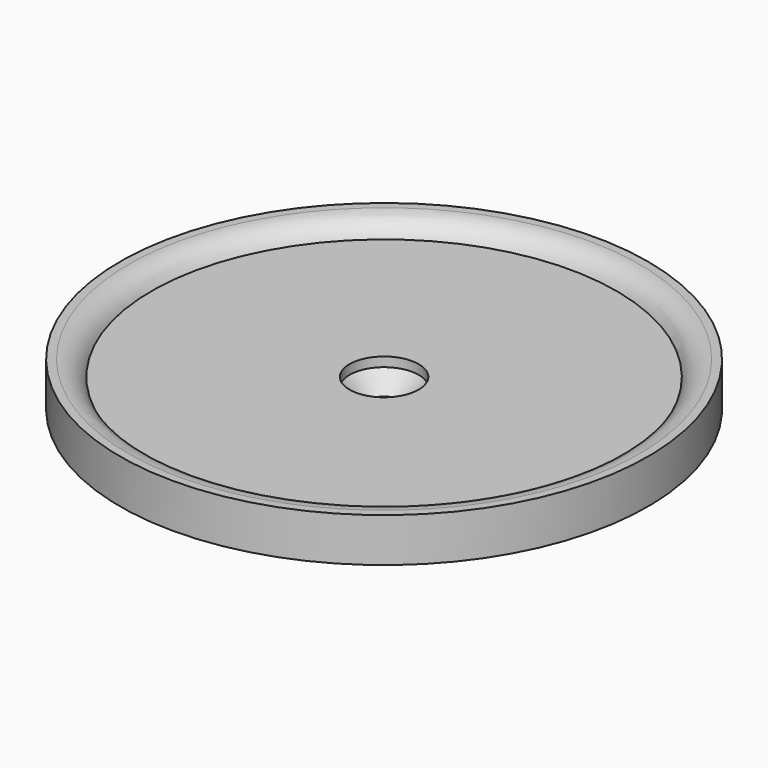
from build123d import *

# Parameters (mm, degrees)
F0_R        = 18.5
F0_R_2      = 1.4
F1_DEPTH    = 2.25
F2_R        = 2.75
F3_DEPTH    = 0.1
F4_S5_R     = 2.75
F4_T6_DEPTH = 6
F6_W        = 2.5
F6_H        = 3.5


# Not quite as in the source:
# - a fillet or chamfer that OpenCascade refuses, or shapes differently, is made with other operations: its cross-section is extruded or revolved along the edge and cut away or added
# - a feature names something its author has since deleted; it is built from what else it names


with BuildPart() as f1:
    # F0 (on Top) → F1 (new body)
    with BuildSketch(Plane.XY):
        Circle(F0_R)
        Circle(F0_R_2, mode=Mode.SUBTRACT)
    extrude(amount=F1_DEPTH)

    # F2 (on face) → F3 (cut)
    with BuildSketch(Plane.XY.offset(2.25)):
        Circle(F2_R)
    extrude(amount=-F3_DEPTH, mode=Mode.SUBTRACT)

    # F4: chamfer of 2 on 1 edges, made by hand


with BuildPart() as f4_tool2:
    # F4_s3 → F4_t4 (revolve)
    with BuildSketch(Plane.XZ):
        Polygon((1.4, 0.15), (3.4, 2.15), (1.4, 2.15), align=None)
    revolve(axis=Axis((0, 0, 2.15), (0, 0, -1)))

    # F4_s5 → F4_t6 (intersect, symmetric)
    with BuildSketch(Plane.XY.offset(1.2)):
        Circle(F4_S5_R)
    extrude(amount=F4_T6_DEPTH, both=True, mode=Mode.INTERSECT)


with BuildPart() as f1_1:
    add(f1.part)

    # F4_t1: cut F4_tool2
    add(f4_tool2.part, mode=Mode.SUBTRACT)

    # F6 (on Right) → F7 (revolve)
    with BuildSketch(Plane.YZ):
        with Locations((-19.75, 1.75)):
            Rectangle(F6_W, F6_H)
    revolve(axis=Axis((0, 0, 7.0907436311), (0, 0, 1)))

    # F8: fillet of radius 2 on 1 edges, made by hand

    # F8_s1 → F8_t2 (revolve, cut)
    with BuildSketch(Plane.YZ):
        with BuildLine():
            ThreePointArc((-20.3540496218, 3.5), (-19.236015633, 3.1583123952), (-18.5, 2.25))
            Line((-18.5, 2.25), (-18.5, 3.5))
            Line((-18.5, 3.5), (-20.3540496218, 3.5))
        make_face()
    revolve(axis=Axis((0, 0, 3.5), (0, 0, 1)), mode=Mode.SUBTRACT)


solid = f1_1.part
